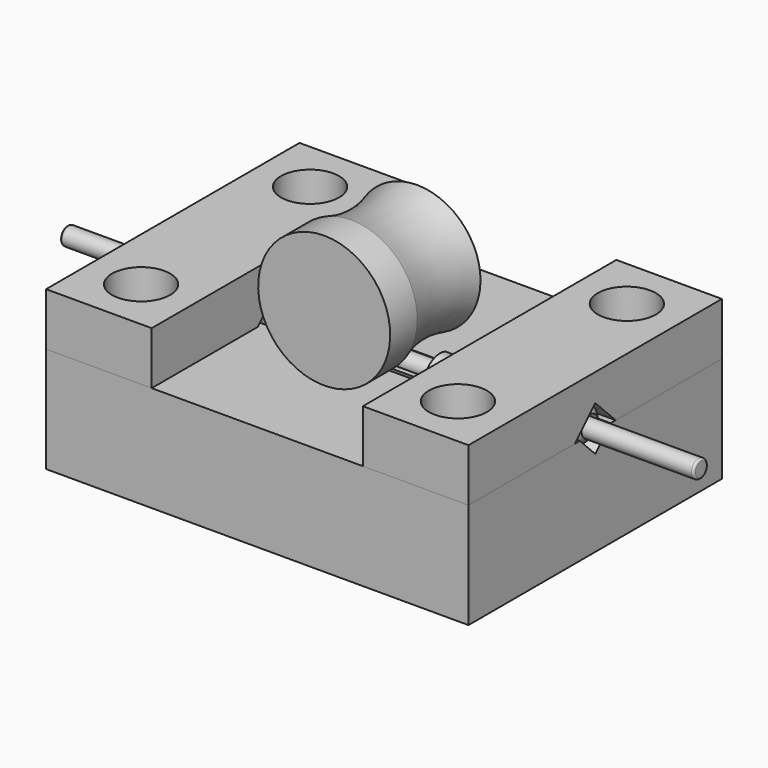
from build123d import *

# Parameters (mm, degrees)
F0_W      = 40
F0_H      = 30
F1_DEPTH  = 10
F4_DEPTH  = 40
F5_D      = 4.2
F7_DEPTH  = 10
F9_DEPTH  = 10
F10_R     = 2.75
F11_DEPTH = 5
F12_R     = 2.75
F13_DEPTH = 5
F15_R     = 1.5
F15_R_2   = 1
F16_DEPTH = 40
F17_W     = 10
F17_H     = 5.7902427018
F18_DEPTH = 25
F20_R     = 0.85
F21_DEPTH = 50
F22_DEPTH = 10
F26_R     = 0.2


# Not quite as in the source:
# - a fillet or chamfer that OpenCascade refuses, or shapes differently, is made with other operations: its cross-section is extruded or revolved along the edge and cut away or added


with BuildPart() as f1:
    # F0 (on Top) → F1 (new body)
    with BuildSketch(Plane.XY):
        with Locations((24.0654195845, -6.8426200747)):
            Rectangle(F0_W, F0_H)
    extrude(amount=F1_DEPTH)

    # F3 (on face) → F4 (cut, through all)
    with BuildSketch(Plane(origin=(4.0654195845, 0, 0), x_dir=(0, -1, 0), z_dir=(-1, 0, 0))):
        with BuildLine():
            ThreePointArc((7.9032802465, 9.2393398282), (6.8426200747, 8.8), (5.781959903, 9.2393398282))
            Line((5.781959903, 9.2393398282), (6.8426200747, 8.1786796564))
            Line((6.8426200747, 8.1786796564), (7.9032802465, 9.2393398282))
        make_face()
        with BuildLine():
            ThreePointArc((5.3729262291, 10), (5.5215130247, 9.5895943677), (5.781959903, 9.2393398282))
            ThreePointArc((5.781959903, 9.2393398282), (6.8426200747, 8.8), (7.9032802465, 9.2393398282))
            ThreePointArc((7.9032802465, 9.2393398282), (8.1637271248, 9.5895943677), (8.3123139204, 10))
            Line((8.3123139204, 10), (6.8426200747, 10))
            Line((6.8426200747, 10), (5.3729262291, 10))
        make_face()
        with BuildLine():
            Line((5.3729262291, 10), (5.0212997312, 10))
            Line((5.0212997312, 10), (5.781959903, 9.2393398282))
            ThreePointArc((5.781959903, 9.2393398282), (5.5215130247, 9.5895943677), (5.3729262291, 10))
        make_face()
        with BuildLine():
            ThreePointArc((8.3123139204, 10), (8.1637271248, 9.5895943677), (7.9032802465, 9.2393398282))
            Line((7.9032802465, 9.2393398282), (8.6639404183, 10))
            Line((8.6639404183, 10), (8.3123139204, 10))
        make_face()
    extrude(amount=-F4_DEPTH, mode=Mode.SUBTRACT)

    # F5 (through all)
    with Locations(Plane.XY.offset(10)):
        with Locations((9.0654195845, 3.1573799253), (39.0654195845, 3.1573799253), (39.0654195845, -16.8426200747), (9.0654195845, -16.8426200747)):
            Hole(F5_D / 2)


with BuildPart() as f7:
    # F6 (on face) → F7 (new body)
    with BuildSketch(Plane(origin=(4.0654195845, 0, 0), x_dir=(0, -1, 0), z_dir=(-1, 0, 0))):
        Polygon((-8.1573799253, 15), (-8.1573799253, 10), (4.4212997312, 10), (5.781959903, 11.3606601718), (6.8426200747, 12.4213203436), (7.9032802476, 11.3606601707), (9.2639404183, 10), (21.8426200747, 10), (21.8426200747, 15), align=None)
    extrude(amount=-F7_DEPTH)

    # F10 (on face) → F11 (cut, through all)
    with BuildSketch(Plane.XY.offset(15)):
        with Locations((9.0654195845, 3.1573799253)):
            Circle(F10_R)
        with Locations((9.0654195845, -16.8426200747)):
            Circle(F10_R)
    extrude(amount=-F11_DEPTH, mode=Mode.SUBTRACT)


with BuildPart() as f9:
    # F8 (on face) → F9 (new body)
    with BuildSketch(Plane.YZ.offset(44.0654195845)):
        Polygon((-6.8426200747, 12.4213203436), (-5.781959903, 11.3606601718), (-4.4212997312, 10), (8.1573799253, 10), (8.1573799253, 15), (-21.8426200747, 15), (-21.8426200747, 10), (-9.2639404183, 10), (-7.9032802476, 11.3606601707), align=None)
    extrude(amount=-F9_DEPTH)

    # F12 (on face) → F13 (cut, through all)
    with BuildSketch(Plane.XY.offset(15)):
        with Locations((39.0654195845, 3.1573799253)):
            Circle(F12_R)
        with Locations((39.0654195845, -16.8426200747)):
            Circle(F12_R)
    extrude(amount=-F13_DEPTH, mode=Mode.SUBTRACT)


with BuildPart() as f16:
    # F15 (on offset) → F16 (new body)
    with BuildSketch(Plane(origin=(4.0654195845, 0, 0), x_dir=(0, -1, 0), z_dir=(-1, 0, 0))):
        with Locations((6.8426200747, 10.3)):
            Circle(F15_R)
        with Locations((6.8426200747, 10.3)):
            Circle(F15_R_2, mode=Mode.SUBTRACT)
    extrude(amount=-F16_DEPTH)

    # F17 (on face) → F18 (cut)
    with BuildSketch(Plane.XZ.offset(21.8426200747)):
        with Locations((24.0654195845, 12.8951213509)):
            Rectangle(F17_W, F17_H)
        Polygon((19.0654195845, 10), (19.0654195845, 15.7902427018), (18.0654195845, 15.7902427018), align=None)
        Polygon((30.0654195845, 15.7902427018), (29.0654195845, 15.7902427018), (29.0654195845, 10), align=None)
    extrude(amount=-F18_DEPTH, mode=Mode.SUBTRACT)

    # F19: chamfer of 1 on 2 edges, made by hand

    # F19_s1 → F19_t2 (revolve, cut)
    with BuildSketch(Plane.XY.offset(10.3)):
        Polygon((5.0654195845, -8.3426200747), (4.0654195845, -7.3426200747), (4.0654195845, -8.3426200747), align=None)
    revolve(axis=Axis((4.0654195845, -6.8426200747, 10.3), (-1, 0, 0)), mode=Mode.SUBTRACT)

    # F19_s3 → F19_t4 (revolve, cut)
    with BuildSketch(Plane.XY.offset(10.3)):
        Polygon((43.0654195845, -8.3426200747), (44.0654195845, -7.3426200747), (44.0654195845, -8.3426200747), align=None)
    revolve(axis=Axis((44.0654195845, -6.8426200747, 10.3), (-1, 0, 0)), mode=Mode.SUBTRACT)


with BuildPart() as f21:
    # F20 (on offset) → F21 (new body)
    with BuildSketch(Plane(origin=(4.0654195845, 0, 0), x_dir=(0, -1, 0), z_dir=(-1, 0, 0))):
        with Locations((6.8426200747, 10.15)):
            Circle(F20_R)
    extrude(amount=-F21_DEPTH)

    # F22 (add): a face of the model
    f22_faces = [f21.faces().sort_by_distance(p)[0] for p in [
        (4.0654195845, -6.8426200747, 10.15),
    ]]
    extrude(f22_faces, amount=F22_DEPTH)

    # F26
    f26_edges = [f21.edges().sort_by_distance(p)[0] for p in [
        (-5.93458, -5.99262, 10.15),
        (54.06542, -5.99262, 10.15),
    ]]
    fillet(f26_edges, radius=F26_R)


with BuildPart() as f25:
    # F24 (on offset) → F25 (revolve)
    with BuildSketch(Plane(origin=(24.0654195845, 0, 0), x_dir=(0, -1, 0), z_dir=(-1, 0, 0))):
        with BuildLine():
            Line((13.9225880235, 16.5), (13.9225880235, 22.75))
            Line((13.9225880235, 22.75), (10.7225880235, 22.75))
            ThreePointArc((10.7225880235, 22.75), (6.8426200747, 22), (2.9225880235, 22.5))
            Line((2.9225880235, 22.5), (2.9225880235, 21.7202004913))
            Line((2.9225880235, 21.7202004913), (2.9225880235, 16.5))
            Line((2.9225880235, 16.5), (13.9225880235, 16.5))
        make_face()
    revolve(axis=Axis((24.0654195845, -8.4225880235, 16.5), (0, -1, 0)))


solid = Compound([f1.part, f7.part, f9.part, f16.part, f21.part, f25.part])
